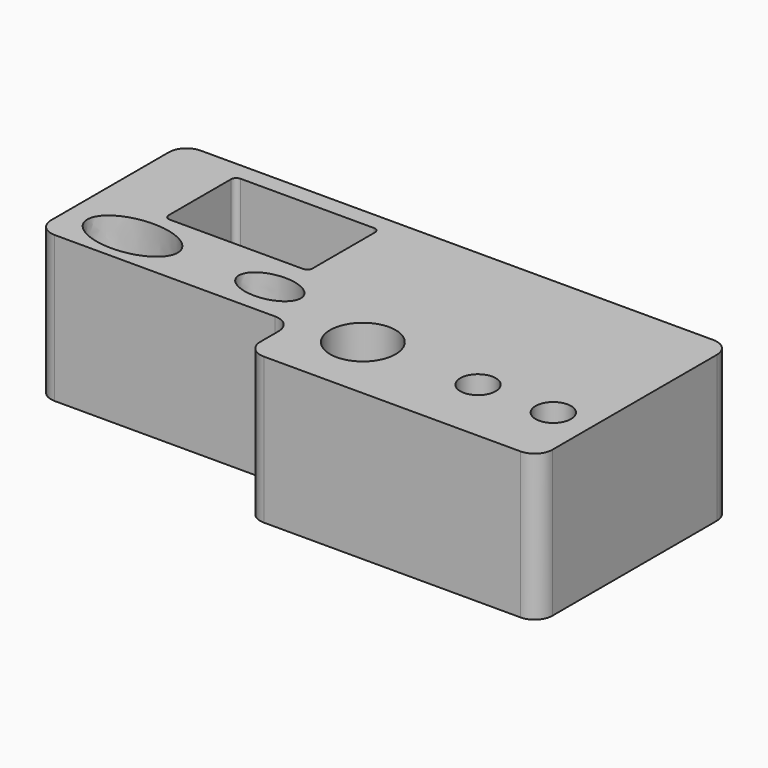
from build123d import *

# Parameters (mm, degrees)
F0_W      = 157.1625
F0_H      = 52.3875
F0_W_2    = 41.275
F0_H_2    = 25.4
F1_DEPTH  = 33.02
F2_W      = 73.025
F2_H      = 52.3875
F3_DEPTH  = 8.89
F4_R      = 5.08
F5_R      = 1.524
F7_W      = 83.75197649
F7_H      = 69.1601932049
F8_DEPTH  = 33.02
F9_DEPTH  = 8.89
F10_R     = 9.398
F10_R_2   = 5.08
F11_DEPTH = 50.8
F12_R     = 5.08


# Not quite as in the source:
# - a feature of the source that left no trace in its solid (it failed there, or was rolled back) is left out


with BuildPart() as f1:
    # F0 (on Top) → F1 (new body)
    with BuildSketch(Plane.XY):
        with Locations((78.58125, -26.19375)):
            Rectangle(F0_W, F0_H)
        with BuildLine():
            add(Edge.make_bspline(
                [(32.004, -41.91), (32.004, -28.8217580726), (12.573, -35.3658790363), (-6.858, -41.91), (12.573, -48.4541209637), (32.004, -54.9982419274), (32.004, -41.91)],
                knots=[0, 0, 0, 2.0943951024, 2.0943951024, 4.1887902048, 4.1887902048, 6.2831853072, 6.2831853072, 6.2831853072], degree=2, weights=[1, 0.5, 1, 0.5, 1, 0.5, 1]))
        make_face(mode=Mode.SUBTRACT)
        with BuildLine():
            add(Edge.make_bspline(
                [(67.31, -41.91), (67.31, -32.3192882683), (53.975, -37.1146441342), (40.64, -41.91), (53.975, -46.7053558658), (67.31, -51.5007117317), (67.31, -41.91)],
                knots=[0, 0, 0, 2.0943951024, 2.0943951024, 4.1887902048, 4.1887902048, 6.2831853072, 6.2831853072, 6.2831853072], degree=2, weights=[1, 0.5, 1, 0.5, 1, 0.5, 1]))
        make_face(mode=Mode.SUBTRACT)
        with Locations((39.6875, -17.78)):
            Rectangle(F0_W_2, F0_H_2, mode=Mode.SUBTRACT)
    extrude(amount=F1_DEPTH)

    # F2 (on Top) → F3 (join)
    with BuildSketch(Plane.XY):
        with Locations((36.5125, -26.19375)):
            Rectangle(F2_W, F2_H)
    extrude(amount=-F3_DEPTH)

    # F4
    f4_edges = [f1.edges().sort_by_distance(p)[0] for p in [
        (73.025, -52.3875, -4.445),
        (157.1625, 0, 16.51),
        (0, 0, 12.065),
        (0, -52.3875, 12.065),
    ]]
    fillet(f4_edges, radius=F4_R)

    # F5
    f5_edges = [f1.edges().sort_by_distance(p)[0] for p in [
        (19.05, -5.08, 16.51),
        (19.05, -30.48, 16.51),
        (60.325, -30.48, 16.51),
        (60.325, -5.08, 16.51),
    ]]
    fillet(f5_edges, radius=F5_R)

    # F7 (on Top) → F8 (join)
    with BuildSketch(Plane.XY):
        with Locations((115.2868717909, -34.5800966024)):
            Rectangle(F7_W, F7_H)
    extrude(amount=F8_DEPTH)

    # F9 (add): a face of the model
    f9_faces = [f1.faces().sort_by_distance(p)[0] for p in [
        (115.0993902801, -34.5668277536, 0),
    ]]
    extrude(f9_faces, amount=F9_DEPTH)

    # F10 (on face) → F11 (cut)
    with BuildSketch(Plane.XY.offset(33.02)):
        with Locations((91.44, -49.8475)):
            Circle(F10_R)
        with Locations((124.46, -49.8475)):
            Circle(F10_R_2)
        with Locations((146.05, -49.8475)):
            Circle(F10_R_2)
    extrude(amount=-F11_DEPTH, mode=Mode.SUBTRACT)

    # F12
    f12_edges = [f1.edges().sort_by_distance(p)[0] for p in [
        (73.410884, -52.3875, 12.065),
        (73.410884, -69.160193, 12.065),
        (157.16286, -69.160193, 12.065),
        (157.16286, 0, 12.065),
    ]]
    fillet(f12_edges, radius=F12_R)


solid = f1.part
